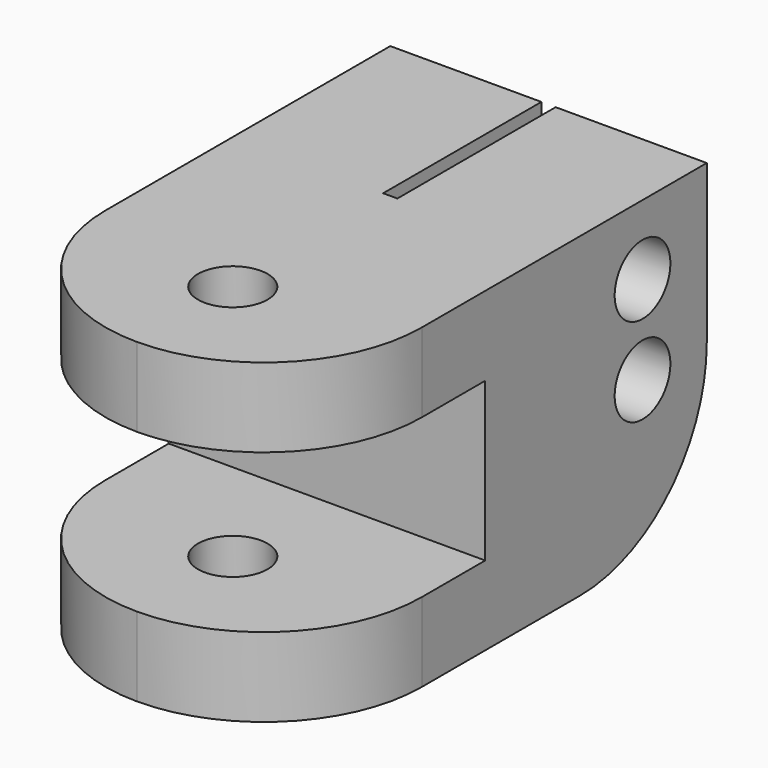
from build123d import *

# Parameters (mm, degrees)
F0_W      = 10.16
F0_H      = 10.16
F1_DEPTH  = 10.16
F2_T      = -2.54
F3_W      = 10.16
F3_H      = 10.16
F4_DEPTH  = 6.35
F5_R      = 1.1176
F6_DEPTH  = 10.16
F7_R      = 1.1176
F8_DEPTH  = 10.16
F9_R      = 5.07999
F10_W     = 0.4572
F10_H     = 6.35
F11_DEPTH = 3.6068


# Not quite as in the source:
# - a fillet or chamfer is up to 0.001 mm smaller than in the source, because OpenCascade refuses the exact size


with BuildPart() as f1:
    # F0 (on Front) → F1 (new body)
    with BuildSketch(Plane.XZ):
        Rectangle(F0_W, F0_H)
    extrude(amount=F1_DEPTH)

    # F2
    f2_openings = [f1.faces().sort_by_distance(p)[0] for p in [
        (0, -10.16, 0),
        (5.08, -5.08, 0),
        (-5.08, -5.08, 0),
    ]]
    offset(amount=F2_T, openings=f2_openings)

    # F3 (on face) → F4 (join)
    with BuildSketch(Plane(origin=(0, 0, 0), x_dir=(-1, 0, 0), z_dir=(0, 1, 0))):
        Rectangle(F3_W, F3_H)
    extrude(amount=F4_DEPTH)

    # F5 (on face) → F6 (cut)
    with BuildSketch(Plane.YZ.offset(5.08)):
        with Locations((3.7731814664, 0)):
            Circle(F5_R)
        with Locations((3.7731814664, 2.838186454)):
            Circle(F5_R)
    extrude(amount=-F6_DEPTH, mode=Mode.SUBTRACT)

    # F7 (on face) → F8 (cut)
    with BuildSketch(Plane.XY.offset(5.08)):
        with Locations((0, -6.3200981603)):
            Circle(F7_R)
    extrude(amount=-F8_DEPTH, mode=Mode.SUBTRACT)

    # F9 (radius 5.08 in the source; OpenCascade refuses exactly that, so slightly less here)
    f9_edges = [f1.edges().sort_by_distance(p)[0] for p in [
        (5.08, -10.16, -3.81),
        (5.08, -10.16, 3.81),
        (-5.08, -10.16, 3.81),
        (-5.08, -10.16, -3.81),
        (0, 6.35, -5.08),
    ]]
    fillet(f9_edges, radius=F9_R)

    # F10 (on face) → F11 (cut)
    with BuildSketch(Plane.XY.offset(5.08)):
        with Locations((0, 3.175)):
            Rectangle(F10_W, F10_H)
    extrude(amount=-F11_DEPTH, mode=Mode.SUBTRACT)


solid = f1.part
